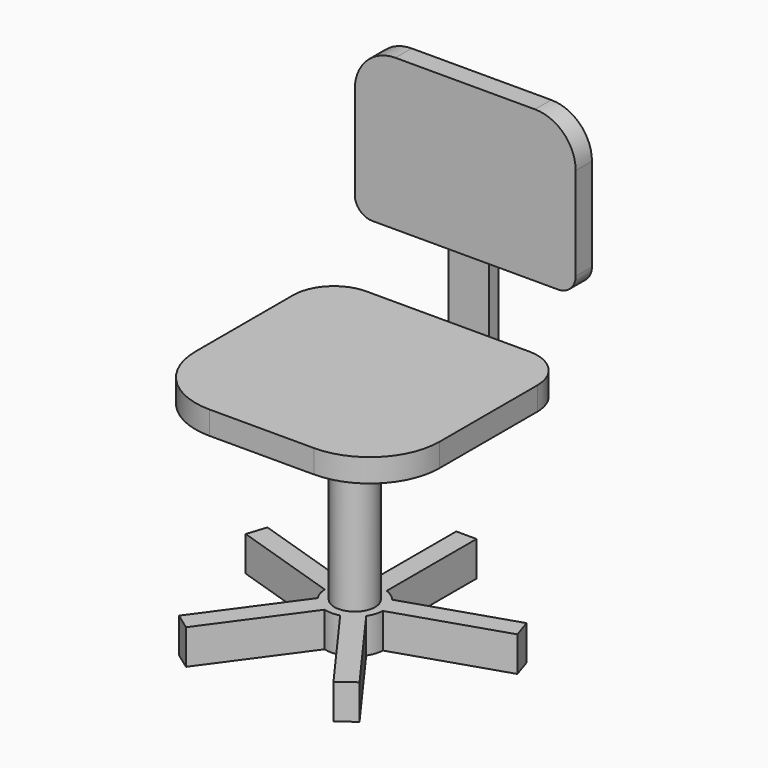
from build123d import *

# Parameters (mm, degrees)
F1_DEPTH  = 60
F2_R      = 35
F3_DEPTH  = 300
F4_W      = 420
F4_H      = 400
F5_DEPTH  = 40
F6_R      = 120
F7_R      = 70
F8_W      = 70
F8_H      = 20
F11_W     = 35
F11_H     = 260
F12_DEPTH = 190
F13_R     = 70
F14_R     = 30


with BuildPart() as f1:
    # F0 (on Top) → F1 (new body)
    with BuildSketch(Plane.XY):
        with BuildLine():
            Line((-233.6613613124, 57.5205896148), (-49.9528927063, -2.1699102001))
            ThreePointArc((-49.9528927063, -2.1699102001), (-47.5528258148, -15.4508497187), (-41.688180332, -27.6060794139))
            Line((-41.688180332, -27.6060794139), (-155.2262579518, -183.8778367349))
            Line((-155.2262579518, -183.8778367349), (-126.9106631486, -204.4503205651))
            Line((-126.9106631486, -204.4503205651), (-13.3725855288, -48.1785632442))
            ThreePointArc((-13.3725855288, -48.1785632442), (0, -50), (13.3725855288, -48.1785632442))
            Line((13.3725855288, -48.1785632442), (126.9106631486, -204.4503205651))
            Line((126.9106631486, -204.4503205651), (155.2262579518, -183.8778367349))
            Line((155.2262579518, -183.8778367349), (41.688180332, -27.6060794139))
            ThreePointArc((41.688180332, -27.6060794139), (47.5528258148, -15.4508497187), (49.9528927063, -2.1699102001))
            Line((49.9528927063, -2.1699102001), (233.6613613124, 57.5205896148))
            Line((233.6613613124, 57.5205896148), (222.8457665093, 90.8075676852))
            Line((222.8457665093, 90.8075676852), (39.1372979031, 31.1170678702))
            ThreePointArc((39.1372979031, 31.1170678702), (29.3892626146, 40.4508497187), (17.5, 46.837484988))
            Line((17.5, 46.837484988), (17.5, 240))
            Line((17.5, 240), (-17.5, 240))
            Line((-17.5, 240), (-17.5, 46.837484988))
            ThreePointArc((-17.5, 46.837484988), (-29.3892626146, 40.4508497187), (-39.1372979031, 31.1170678702))
            Line((-39.1372979031, 31.1170678702), (-222.8457665093, 90.8075676852))
            Line((-222.8457665093, 90.8075676852), (-233.6613613124, 57.5205896148))
        make_face()
    extrude(amount=F1_DEPTH)

    # F2 (on face) → F3 (join)
    with BuildSketch(Plane.XY.offset(60)):
        Circle(F2_R)
    extrude(amount=F3_DEPTH)


with BuildPart() as f5:
    # F4 (on face) → F5 (new body)
    with BuildSketch(Plane.XY.offset(360)):
        Rectangle(F4_W, F4_H)
    extrude(amount=F5_DEPTH)

    # F6
    f6_edges = [f5.edges().sort_by_distance(p)[0] for p in [
        (210, -200, 380),
        (-210, -200, 380),
    ]]
    fillet(f6_edges, radius=F6_R)

    # F7
    f7_edges = [f5.edges().sort_by_distance(p)[0] for p in [
        (210, 200, 380),
        (-210, 200, 380),
    ]]
    fillet(f7_edges, radius=F7_R)


with BuildPart() as f10:
    # F10: sweep along a path in F9
    with BuildLine(Plane.YZ) as f10_path:
        Line((0, 315), (230, 315))
        ThreePointArc((230, 315), (251.2132034356, 323.7867965644), (260, 345))
        Line((260, 345), (260, 485))
    # F8 (on Front) → F10 (sweep)
    with BuildSketch(Plane.XZ):
        with Locations((0, 320)):
            Rectangle(F8_W, F8_H)
    sweep(path=f10_path.line)

    # F11 (on Right) → F12 (join, symmetric)
    with BuildSketch(Plane.YZ):
        with Locations((255, 615)):
            Rectangle(F11_W, F11_H)
    extrude(amount=F12_DEPTH, both=True)

    # F13
    f13_edges = [f10.edges().sort_by_distance(p)[0] for p in [
        (190, 255, 745),
        (-190, 255, 745),
    ]]
    fillet(f13_edges, radius=F13_R)

    # F14
    f14_edges = [f10.edges().sort_by_distance(p)[0] for p in [
        (-190, 255, 485),
        (190, 255, 485),
    ]]
    fillet(f14_edges, radius=F14_R)


solid = Compound([f1.part, f5.part, f10.part])
